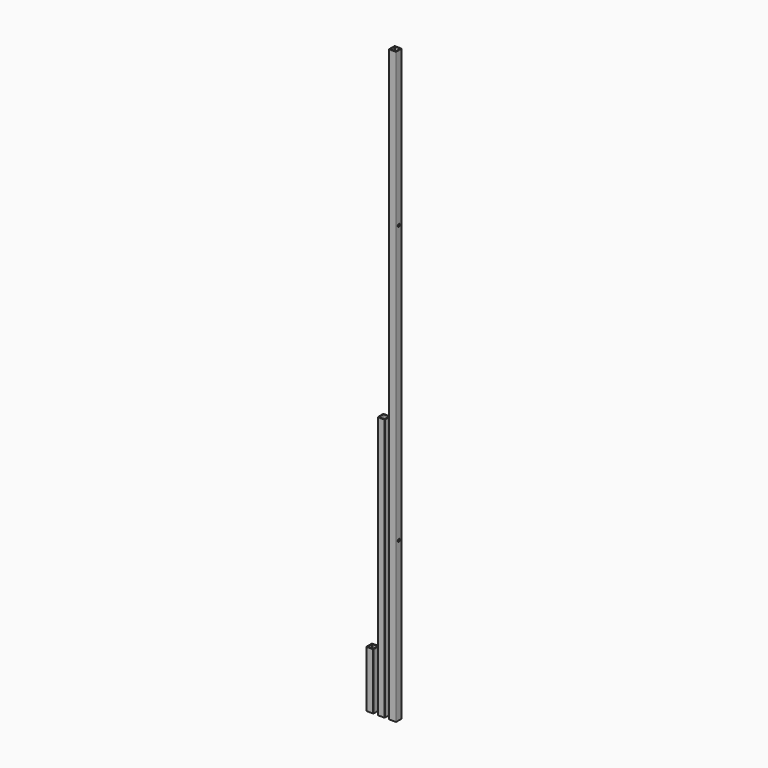
from build123d import *

# Parameters (mm, degrees)
F1_DEPTH = 508
F2_DEPTH = 2355.85
F3_DEPTH = 5295.9
F6_R     = 12.7
F7_DEPTH = 266.701


with BuildPart() as f1:
    # F0 (on Top) → F1 (new body)
    with BuildSketch(Plane.XY):
        with BuildLine():
            ThreePointArc((31.75, 28.575), (30.8200640303, 30.8200640303), (28.575, 31.75))
            Line((28.575, 31.75), (-28.575, 31.75))
            ThreePointArc((-28.575, 31.75), (-30.8200640303, 30.8200640303), (-31.75, 28.575))
            Line((-31.75, 28.575), (-31.75, -28.575))
            ThreePointArc((-31.75, -28.575), (-30.8200640303, -30.8200640303), (-28.575, -31.75))
            Line((-28.575, -31.75), (28.575, -31.75))
            ThreePointArc((28.575, -31.75), (30.8200640303, -30.8200640303), (31.75, -28.575))
            Line((31.75, -28.575), (31.75, 28.575))
        make_face()
        with BuildLine():
            Line((-22.225, 25.4), (22.225, 25.4))
            ThreePointArc((22.225, 25.4), (24.4700640303, 24.4700640303), (25.4, 22.225))
            Line((25.4, 22.225), (25.4, -22.225))
            ThreePointArc((25.4, -22.225), (24.4700640303, -24.4700640303), (22.225, -25.4))
            Line((22.225, -25.4), (-22.225, -25.4))
            ThreePointArc((-22.225, -25.4), (-24.4700640303, -24.4700640303), (-25.4, -22.225))
            Line((-25.4, -22.225), (-25.4, 22.225))
            ThreePointArc((-25.4, 22.225), (-24.4700640303, 24.4700640303), (-22.225, 25.4))
        make_face(mode=Mode.SUBTRACT)
    extrude(amount=F1_DEPTH)


with BuildPart() as f2:
    # F0 (on Top) → F2 (new body)
    with BuildSketch(Plane.XY):
        with BuildLine():
            Line((73.025, -31.75), (130.175, -31.75))
            ThreePointArc((130.175, -31.75), (132.4200640303, -30.8200640303), (133.35, -28.575))
            Line((133.35, -28.575), (133.35, 28.575))
            ThreePointArc((133.35, 28.575), (132.4200640303, 30.8200640303), (130.175, 31.75))
            Line((130.175, 31.75), (73.025, 31.75))
            ThreePointArc((73.025, 31.75), (70.7799359697, 30.8200640303), (69.85, 28.575))
            Line((69.85, 28.575), (69.85, -28.575))
            ThreePointArc((69.85, -28.575), (70.7799359697, -30.8200640303), (73.025, -31.75))
        make_face()
        with BuildLine():
            Line((79.375, 25.4), (123.825, 25.4))
            ThreePointArc((123.825, 25.4), (126.0700640303, 24.4700640303), (127, 22.225))
            Line((127, 22.225), (127, -22.225))
            ThreePointArc((127, -22.225), (126.0700640303, -24.4700640303), (123.825, -25.4))
            Line((123.825, -25.4), (79.375, -25.4))
            ThreePointArc((79.375, -25.4), (77.1299359697, -24.4700640303), (76.2, -22.225))
            Line((76.2, -22.225), (76.2, 22.225))
            ThreePointArc((76.2, 22.225), (77.1299359697, 24.4700640303), (79.375, 25.4))
        make_face(mode=Mode.SUBTRACT)
    extrude(amount=F2_DEPTH)


with BuildPart() as f3:
    # F0 (on Top) → F3 (new body)
    with BuildSketch(Plane.XY):
        with BuildLine():
            Line((174.625, -31.75), (231.775, -31.75))
            ThreePointArc((231.775, -31.75), (234.0200640303, -30.8200640303), (234.95, -28.575))
            Line((234.95, -28.575), (234.95, 28.575))
            ThreePointArc((234.95, 28.575), (234.0200640303, 30.8200640303), (231.775, 31.75))
            Line((231.775, 31.75), (174.625, 31.75))
            ThreePointArc((174.625, 31.75), (172.3799359697, 30.8200640303), (171.45, 28.575))
            Line((171.45, 28.575), (171.45, -28.575))
            ThreePointArc((171.45, -28.575), (172.3799359697, -30.8200640303), (174.625, -31.75))
        make_face()
        with BuildLine():
            Line((180.975, 25.4), (225.425, 25.4))
            ThreePointArc((225.425, 25.4), (227.6700640303, 24.4700640303), (228.6, 22.225))
            Line((228.6, 22.225), (228.6, -22.225))
            ThreePointArc((228.6, -22.225), (227.6700640303, -24.4700640303), (225.425, -25.4))
            Line((225.425, -25.4), (180.975, -25.4))
            ThreePointArc((180.975, -25.4), (178.7299359697, -24.4700640303), (177.8, -22.225))
            Line((177.8, -22.225), (177.8, 22.225))
            ThreePointArc((177.8, 22.225), (178.7299359697, 24.4700640303), (180.975, 25.4))
        make_face(mode=Mode.SUBTRACT)
    extrude(amount=F3_DEPTH)

    # F6 (on face) → F7 (cut, through all)
    with BuildSketch(Plane.YZ.offset(234.95)):
        with Locations((0, 3911.6)):
            Circle(F6_R)
        with Locations((0, 1422.4)):
            Circle(F6_R)
    extrude(amount=-F7_DEPTH, mode=Mode.SUBTRACT)


solid = Compound([f1.part, f2.part, f3.part])
